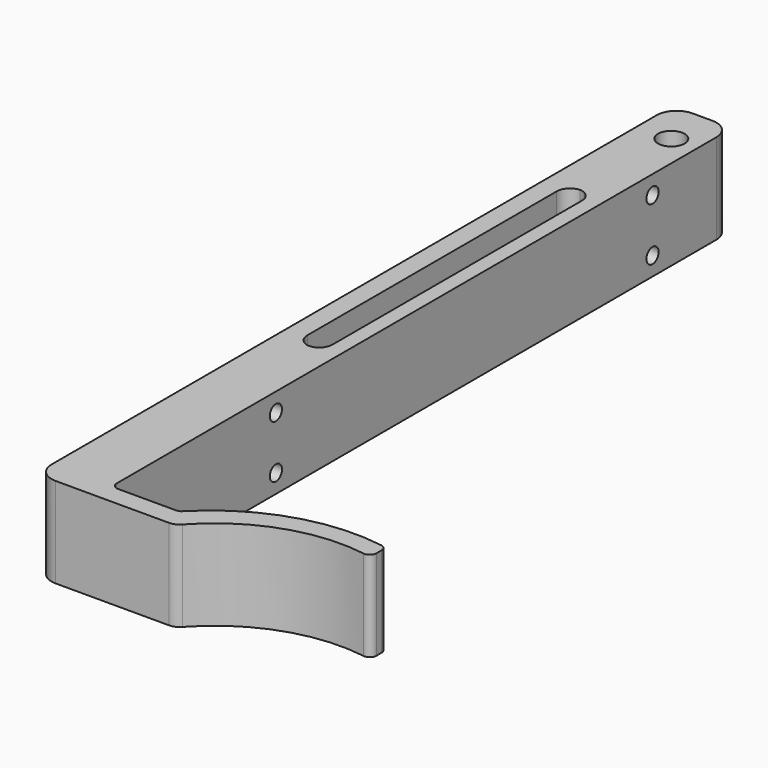
from build123d import *

# Parameters (mm, degrees)
F0_W          = 6
F0_H          = 120
F1_DEPTH      = 12.8
F1_DEPTH_BACK = 0.8
F2_R          = 2
F3_R          = 1
F4_R          = 1.15
F5_DEPTH      = 15
F6_W          = 3.8
F6_H          = 51
F6_R          = 2
F7_DEPTH      = 19
F8_R          = 3
F9_T1_DEPTH   = 13.6


# Not quite as in the source:
# - a fillet or chamfer that OpenCascade refuses, or shapes differently, is made with other operations: its cross-section is extruded or revolved along the edge and cut away or added


with BuildPart() as f1:
    # F0 (on Top) → F1 (new body, two sides)
    with BuildSketch(Plane.XY) as f1_sk:
        Polygon((2.9121718865, 60.9107007086), (-0.0878281135, 60.9107007086), (-0.0878281135, -59.0892992914), (2.9121718865, -59.0892992914), (2.9121718865, -56.0892992914), align=None)
        with Locations((-3.0878281135, 0.9107007086)):
            Rectangle(F0_W, F0_H)
        with BuildLine():
            Line((13.1121718865, -56.0892992914), (2.9121718865, -56.0892992914))
            Line((2.9121718865, -56.0892992914), (2.9121718865, -59.0892992914))
            Line((2.9121718865, -59.0892992914), (14.9121718865, -59.0892992914))
            ThreePointArc((14.9121718865, -59.0892992914), (25.3098855946, -51.9202262022), (37.9121718865, -51.0892992914))
            Line((37.9121718865, -51.0892992914), (37.9121718865, -48.0892992914))
            ThreePointArc((37.9121718865, -48.0892992914), (24.4865924683, -48.9100030948), (13.1121718865, -56.0892992914))
        make_face()
    extrude(amount=-F1_DEPTH)
    extrude(f1_sk.sketch, amount=F1_DEPTH_BACK)

    # F2
    f2_edges = [f1.edges().sort_by_distance(p)[0] for p in [
        (14.912172, -59.089299, -6),
    ]]
    fillet(f2_edges, radius=F2_R)

    # F3
    f3_edges = [f1.edges().sort_by_distance(p)[0] for p in [
        (2.912172, -56.089299, -6),
        (13.112172, -56.089299, -6),
        (37.912172, -48.089299, -6),
        (37.912172, -51.089299, -6),
    ]]
    fillet(f3_edges, radius=F3_R)

    # F4 (on face) → F5 (cut)
    with BuildSketch(Plane.YZ.offset(2.9121718865)):
        with Locations((-25.0892992914, -2)):
            Circle(F4_R)
        with Locations((-25.0892992914, -10)):
            Circle(F4_R)
        with Locations((45.8816848695, -2)):
            Circle(F4_R)
        with Locations((45.8816848695, -10)):
            Circle(F4_R)
    extrude(amount=-F5_DEPTH, mode=Mode.SUBTRACT)

    # F6 (on face) → F7 (cut)
    with BuildSketch(Plane.XY.offset(0.8)):
        with Locations((-1.25, 11.9107007086)):
            Rectangle(F6_W, F6_H)
        with Locations((-1, 54.3107017875)):
            Circle(F6_R)
    extrude(amount=-F7_DEPTH, mode=Mode.SUBTRACT)

    # F8
    f8_edges = [f1.edges().sort_by_distance(p)[0] for p in [
        (-6.087828, 60.910701, -6),
        (2.912172, 60.910701, -6),
        (-6.087828, -59.089299, -6),
    ]]
    fillet(f8_edges, radius=F8_R)

    # F9: fillet of radius 2 on 4 edges, made by hand

    # F9_s2 → F9_t1 (join)
    with BuildSketch(Plane.XY.offset(-12.8)):
        with BuildLine():
            ThreePointArc((-1.15, 37.4107007086), (-2.5642135624, 36.824914271), (-3.15, 35.4107007086))
            Line((-3.15, 35.4107007086), (-3.15, 37.4107007086))
            Line((-3.15, 37.4107007086), (-1.15, 37.4107007086))
        make_face()
        with BuildLine():
            ThreePointArc((0.65, 35.4107007086), (0.0642135624, 36.824914271), (-1.35, 37.4107007086))
            Line((-1.35, 37.4107007086), (0.65, 37.4107007086))
            Line((0.65, 37.4107007086), (0.65, 35.4107007086))
        make_face()
        with BuildLine():
            ThreePointArc((-3.15, -11.5892992914), (-2.5642135624, -13.0035128537), (-1.15, -13.5892992914))
            Line((-1.15, -13.5892992914), (-3.15, -13.5892992914))
            Line((-3.15, -13.5892992914), (-3.15, -11.5892992914))
        make_face()
        with BuildLine():
            ThreePointArc((0.65, -11.5892992914), (0.0642135624, -13.0035128537), (-1.35, -13.5892992914))
            Line((-1.35, -13.5892992914), (0.65, -13.5892992914))
            Line((0.65, -13.5892992914), (0.65, -11.5892992914))
        make_face()
    extrude(amount=F9_T1_DEPTH)


solid = f1.part
